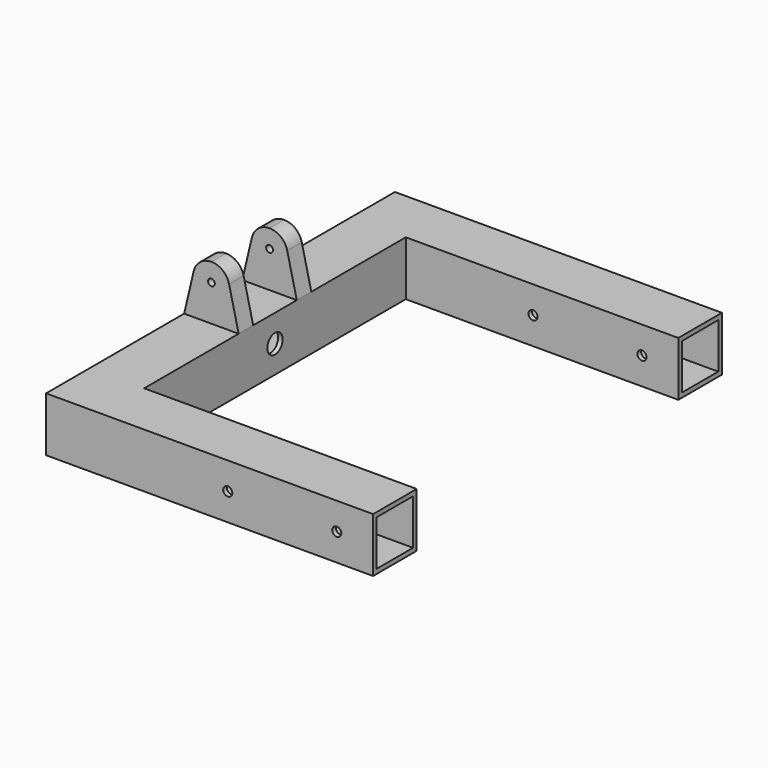
from build123d import *

# Parameters (mm, degrees)
F1_DEPTH = 76.2
F2_T     = -6.35
F4_D     = 12.7
F7_DEPTH = 12.7
F8_R     = 13.4197326433
F9_DEPTH = 228.601


# Not quite as in the source:
# - a feature names something its author has since deleted; it is built from what else it names


with BuildPart() as f1:
    # F0 (on Top) → F1 (new body)
    with BuildSketch(Plane.XY):
        Polygon((-228.6, 304.8), (-228.6, -304.8), (228.6, -304.8), (228.6, -228.6), (-152.4, -228.6), (-152.4, 228.6), (228.6, 228.6), (228.6, 304.8), align=None)
    extrude(amount=F1_DEPTH)

    # F2
    f2_openings = [f1.faces().sort_by_distance(p)[0] for p in [
        (228.6, -266.7, 38.1),
        (228.6, 266.7, 38.1),
    ]]
    offset(amount=F2_T, openings=f2_openings, kind=Kind.INTERSECTION)

    # F4 (through all)
    with Locations(Plane(origin=(0, 304.8, 0), x_dir=(-1, 0, 0), z_dir=(0, 1, 0))):
        with Locations((-177.8, 38.1), (-25.4, 38.1)):
            Hole(F4_D / 2)

    # F6 (on offset) → F7 (join, symmetric)
    with BuildSketch(Plane.XZ.offset(50.8)):
        with BuildLine():
            Line((-215.2195876243, 132.8396907182), (-228.6, 76.2))
            Line((-228.6, 76.2), (-190.5, 76.2))
            Line((-190.5, 76.2), (-190.5, 122.2375))
            ThreePointArc((-190.5, 122.2375), (-195.2625, 127), (-190.5, 131.7625))
            Line((-190.5, 131.7625), (-190.5, 152.4))
            ThreePointArc((-190.5, 152.4), (-206.2612159391, 146.9184354838), (-215.2195876243, 132.8396907182))
        make_face()
        with BuildLine():
            Line((-190.5, 122.2375), (-190.5, 76.2))
            Line((-190.5, 76.2), (-152.4, 76.2))
            Line((-152.4, 76.2), (-165.7804123757, 132.8396907182))
            ThreePointArc((-165.7804123757, 132.8396907182), (-174.7387840609, 146.9184354838), (-190.5, 152.4))
            Line((-190.5, 152.4), (-190.5, 131.7625))
            ThreePointArc((-190.5, 131.7625), (-187.1324039546, 130.3675960454), (-185.7375, 127))
            ThreePointArc((-185.7375, 127), (-187.1324039546, 123.6324039546), (-190.5, 122.2375))
        make_face()
    extrude(amount=F7_DEPTH, both=True)

    # F8 (on Right) → F9 (cut, through all)
    with BuildSketch(Plane.YZ):
        with Locations((0, 38.1)):
            Circle(F8_R)
    extrude(amount=-F9_DEPTH, mode=Mode.SUBTRACT)

    # F10: F1 across plane


with BuildPart() as f1_1:
    add(f1.part)
    add(f1.part.mirror(Plane.XZ))


solid = f1_1.part
